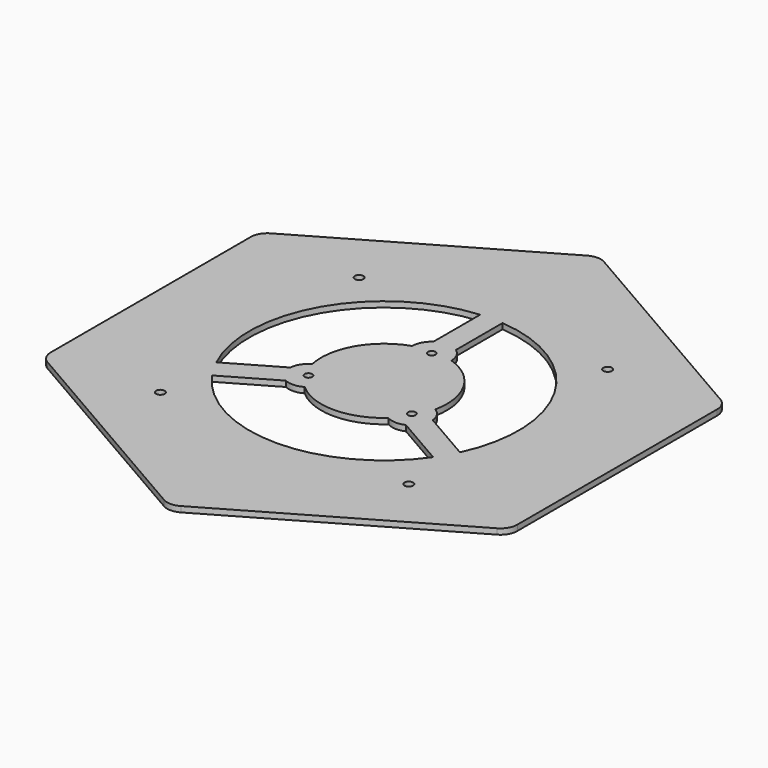
from build123d import *

# Parameters (mm, degrees)
F0_R            = 1.2192
F1_DEPTH        = 1.5875
F2_R            = 1.0922
F3_DEPTH        = 1.5875
F3_COPIES_COUNT = 3
F4_R            = 4.7625


# Not quite as in the source:
# - a pattern or mirror of a feature is missing from the dataset's text; its kind, count and spacing are read off the source's solid


with BuildPart() as f1:
    # F0 (on Top) → F1 (new body)
    with BuildSketch(Plane.XY):
        Polygon((65.9911357684, -38.1), (65.9911357684, 38.1), (0, 76.2), (-65.9911357684, 38.1), (-65.9911357684, -38.1), (0, -76.2), align=None)
        with Locations((-35.1536, -35.1536)):
            Circle(F0_R, mode=Mode.SUBTRACT)
        with Locations((35.1536, -35.1536)):
            Circle(F0_R, mode=Mode.SUBTRACT)
        with Locations((-35.1536, 35.1536)):
            Circle(F0_R, mode=Mode.SUBTRACT)
        with Locations((35.1536, 35.1536)):
            Circle(F0_R, mode=Mode.SUBTRACT)
    extrude(amount=F1_DEPTH)

    # F2 (on face) → F3 (cut, through all)
    with BuildSketch(Plane.XY.offset(1.5875)):
        with BuildLine():
            ThreePointArc((11.8486437632, -13.2566225326), (0, -17.78), (-11.8486437632, -13.2566225326))
            ThreePointArc((-11.8486437632, -13.2566225326), (-14.3916795622, -13.9960432527), (-16.9881251543, -13.4742728402))
            Line((-16.9881251543, -13.4742728402), (-31.2933003438, -21.7333695867))
            ThreePointArc((-31.2933003438, -21.7333695867), (0, -38.1), (31.2933003438, -21.7333695867))
            Line((31.2933003438, -21.7333695867), (16.9881251543, -13.4742728402))
            ThreePointArc((16.9881251543, -13.4742728402), (14.3916795622, -13.9960432527), (11.8486437632, -13.2566225326))
        make_face()
        with Locations((14.6267687632, -8.4447688828)):
            Circle(F2_R)
        with Locations((-14.6267687632, -8.4447688828)):
            Circle(F2_R)
    f3 = extrude(amount=-F3_DEPTH, mode=Mode.SUBTRACT)

    # F3_copies: F3 ×3 about axis
    f3_copies_axis = Axis((0, 0, 0), (0, 0, 1))
    for i in range(1, F3_COPIES_COUNT):
        add(f3.rotate(f3_copies_axis, i * 360 / F3_COPIES_COUNT), mode=Mode.SUBTRACT)

    # F4
    f4_edges = [f1.edges().sort_by_distance(p)[0] for p in [
        (-65.991136, 38.1, 0.79375),
        (0, 76.2, 0.79375),
        (65.991136, 38.1, 0.79375),
        (65.991136, -38.1, 0.79375),
        (0, -76.2, 0.79375),
        (-65.991136, -38.1, 0.79375),
    ]]
    fillet(f4_edges, radius=F4_R)


solid = f1.part
